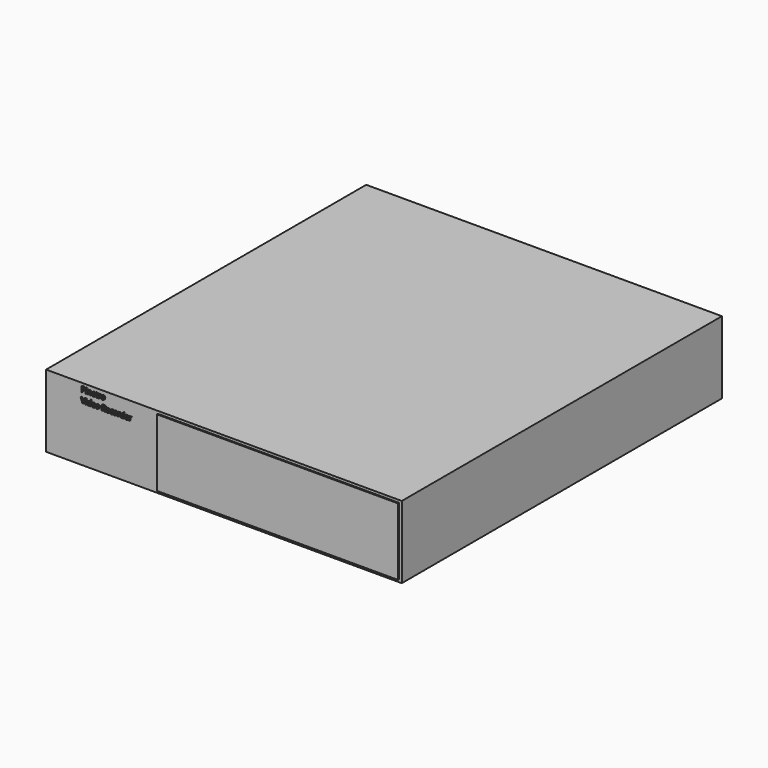
from build123d import *

# Parameters (mm, degrees)
F0_W         = 280
F0_H         = 315
F1_DEPTH     = 57
F2_W         = 190
F2_H         = 53
F2_TEXT_SIZE = 5.5660644011
F3_DEPTH     = 1


# Not quite as in the source:
# - Text() gives the source's letters only with a copy of the font that has no kerning and outlines rounded to 1/6400 em; it was checked with that copy


with BuildPart() as f1:
    # F0 (on Top) → F1 (new body)
    with BuildSketch(Plane.XY):
        with Locations((-140, 157.5)):
            Rectangle(F0_W, F0_H)
    extrude(amount=F1_DEPTH)

    # F2 (on face) → F3 (join)
    with BuildSketch(Plane.XZ):
        with Locations((-97, 28.5)):
            Rectangle(F2_W, F2_H)
        with Locations((-252, 50.9924336312)):
            Text('Pinetro', F2_TEXT_SIZE, font='Open Sans', text_align=(TextAlign.LEFT, TextAlign.BOTTOM))
        with Locations((-252, 43.4225860457)):
            Text('Video Recorder', F2_TEXT_SIZE, font='Open Sans', text_align=(TextAlign.LEFT, TextAlign.BOTTOM))
    extrude(amount=F3_DEPTH)


solid = f1.part
